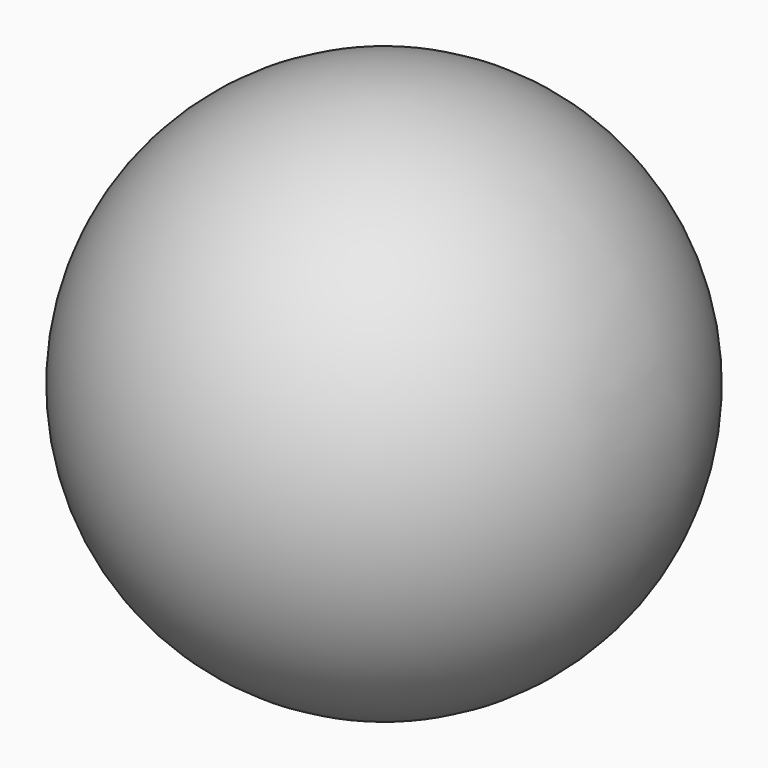
from build123d import *


# Not quite as in the source:
# - the program builds the solid bodies; features that only make, move or delete a surface that nothing else refers to are left out


with BuildPart() as f1:
    # F0 (on Front) → F1 (revolve)
    with BuildSketch(Plane.XZ):
        with BuildLine():
            Line((0, 65.2396578347), (0, 27.1396578347))
            ThreePointArc((0, 27.1396578347), (19.05, 46.1896578347), (0, 65.2396578347))
        make_face()
    revolve(axis=Axis((0, 0, 46.1896578347), (0, 0, 1)))


solid = f1.part
